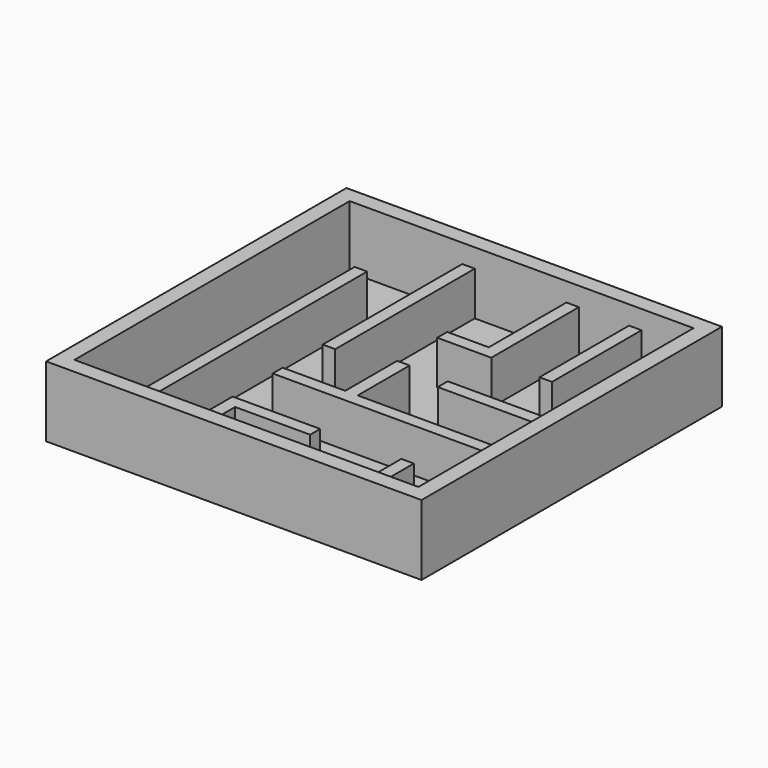
from build123d import *

# Parameters (mm, degrees)
F0_W     = 38.1
F0_H     = 38.1
F1_DEPTH = 0.79375
F2_W     = 38.1
F2_H     = 38.1
F2_W_2   = 34.8996
F2_H_2   = 34.8996
F3_DEPTH = 6.35
F4_W     = 1.27
F4_H     = 17.6995960579
F4_H_2   = 29.188188513
F4_W_2   = 11.795372231
F4_H_3   = 1.27
F4_H_4   = 11.3495960579
F4_H_5   = 5.7700039421
F6_DEPTH = 4.445
F5_R     = 1.27
F7_DEPTH = 0.396875


# Not quite as in the source:
# - a feature names something its author has since deleted; it is built from what else it names


with BuildPart() as f1:
    # F0 (on Top) → F1 (new body)
    with BuildSketch(Plane.XY):
        with Locations((2.218876034, 4.4484467313)):
            Rectangle(F0_W, F0_H)
    extrude(amount=F1_DEPTH)

    # F2 (on face) → F3 (join)
    with BuildSketch(Plane.XY.offset(0.79375)):
        with Locations((2.218876034, 4.4484467313)):
            Rectangle(F2_W, F2_H)
        with Locations((2.218876034, 4.4484467313)):
            Rectangle(F2_W_2, F2_H_2, mode=Mode.SUBTRACT)
    extrude(amount=F3_DEPTH)

    # F4 (on face) → F6 (join)
    with BuildSketch(Plane.XY.offset(0.79375)):
        with Locations((-3.165923966, 13.0484487024)):
            Rectangle(F4_W, F4_H)
        with Locations((-9.515923966, 1.5927409878)):
            Rectangle(F4_W, F4_H_2)
        Polygon((-3.800923966, -2.1513493266), (19.668676034, -2.1513493266), (19.668676034, -0.8813493266), (3.819076034, -0.8813493266), (3.819076034, 5.701588226), (2.549076034, 5.701588226), (2.549076034, -0.8813493266), (-3.800923966, -0.8813493266), align=None)
        Polygon((-3.800923966, -8.5013493266), (-3.800923966, -13.0013532687), (-2.530923966, -13.0013532687), (-2.530923966, -8.5013493266), (5.089076034, -8.5013493266), (5.089076034, -7.2313493266), (3.819076034, -7.2313493266), (-3.800923966, -7.2313493266), align=None)
        Polygon((8.0383015836, 21.8982467313), (6.7683015836, 21.8982467313), (6.7683015836, 12.051588226), (2.549076034, 12.051588226), (2.549076034, 10.781588226), (8.0383015836, 10.781588226), align=None)
        with Locations((13.7709899185, 4.8336506734)):
            Rectangle(F4_W_2, F4_H_3)
        with Locations((13.7533015836, 16.2234487024)):
            Rectangle(F4_W, F4_H_4)
        with Locations((13.953676034, -10.1163512976)):
            Rectangle(F4_W, F4_H_5)
    extrude(amount=F6_DEPTH)

    # F5 (on face) → F7 (cut)
    with BuildSketch(Plane.XY.offset(0.79375)):
        with Locations((17.0904958928, -8.8772866875)):
            Circle(F5_R)
        with Locations((-12.6393535174, -8.3864945918)):
            Circle(F5_R)
    extrude(amount=-F7_DEPTH, mode=Mode.SUBTRACT)


solid = f1.part
